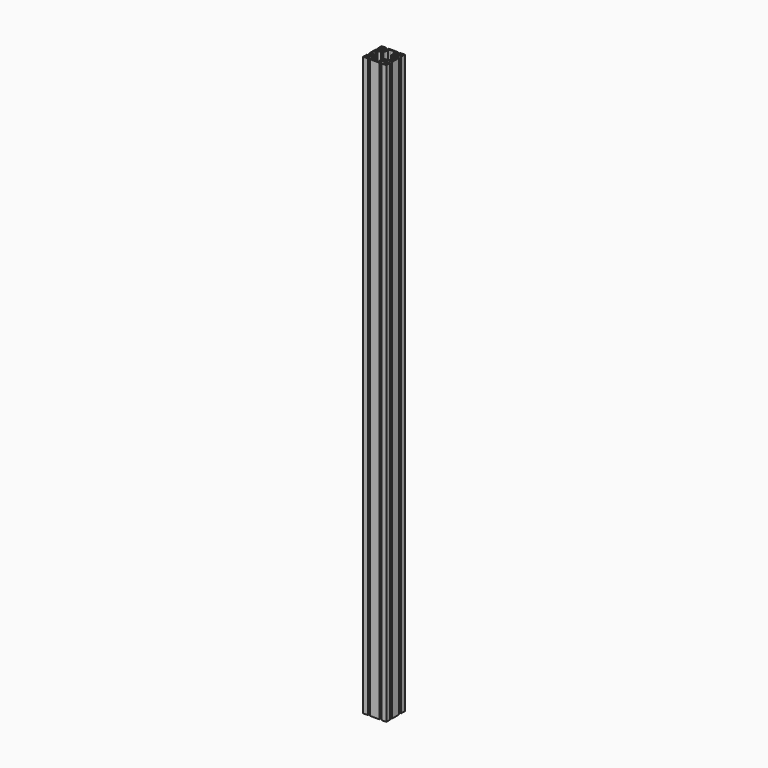
from build123d import *

# Parameters (mm, degrees)
F0_R     = 3
F0_R_2   = 2.5
F1_DEPTH = 1500
F2_R     = 2
F3_R     = 7


# Not quite as in the source:
# - a feature names something its author has since deleted; it is built from what else it names


with BuildPart() as f1:
    # F0 (on Top) → F1 (new body)
    with BuildSketch(Plane.XY):
        with BuildLine():
            Line((18.15, -30), (30, -30))
            Line((30, -30), (30, -18.15))
            Line((30, -18.15), (27.5, -18.15))
            Line((27.5, -18.15), (27.5, -20.15))
            Line((27.5, -20.15), (21.5477069044, -20.15))
            ThreePointArc((21.5477069044, -20.15), (19.5, -15), (21.5477069044, -9.85))
            Line((21.5477069044, -9.85), (27.5, -9.85))
            Line((27.5, -9.85), (27.5, -11.85))
            Line((27.5, -11.85), (30, -11.85))
            Line((30, -11.85), (30, 11.85))
            Line((30, 11.85), (27.5, 11.85))
            Line((27.5, 11.85), (27.5, 9.85))
            Line((27.5, 9.85), (21.5477069044, 9.85))
            ThreePointArc((21.5477069044, 9.85), (19.5, 15), (21.5477069044, 20.15))
            Line((21.5477069044, 20.15), (27.5, 20.15))
            Line((27.5, 20.15), (27.5, 18.15))
            Line((27.5, 18.15), (30, 18.15))
            Line((30, 18.15), (30, 30))
            Line((30, 30), (18.15, 30))
            Line((18.15, 30), (18.15, 27.5))
            Line((18.15, 27.5), (20.15, 27.5))
            Line((20.15, 27.5), (20.15, 21.5477069044))
            ThreePointArc((20.15, 21.5477069044), (15, 19.5), (9.85, 21.5477069044))
            Line((9.85, 21.5477069044), (9.85, 27.5))
            Line((9.85, 27.5), (11.85, 27.5))
            Line((11.85, 27.5), (11.85, 30))
            Line((11.85, 30), (-11.85, 30))
            Line((-11.85, 30), (-11.85, 27.5))
            Line((-11.85, 27.5), (-9.85, 27.5))
            Line((-9.85, 27.5), (-9.85, 21.5477069044))
            ThreePointArc((-9.85, 21.5477069044), (-15, 19.5), (-20.15, 21.5477069044))
            Line((-20.15, 21.5477069044), (-20.15, 27.5))
            Line((-20.15, 27.5), (-18.15, 27.5))
            Line((-18.15, 27.5), (-18.15, 30))
            Line((-18.15, 30), (-30, 30))
            Line((-30, 30), (-30, 18.15))
            Line((-30, 18.15), (-27.5, 18.15))
            Line((-27.5, 18.15), (-27.5, 20.15))
            Line((-27.5, 20.15), (-21.5477069044, 20.15))
            ThreePointArc((-21.5477069044, 20.15), (-19.5, 15), (-21.5477069044, 9.85))
            Line((-21.5477069044, 9.85), (-27.5, 9.85))
            Line((-27.5, 9.85), (-27.5, 11.85))
            Line((-27.5, 11.85), (-30, 11.85))
            Line((-30, 11.85), (-30, -11.85))
            Line((-30, -11.85), (-27.5, -11.85))
            Line((-27.5, -11.85), (-27.5, -9.85))
            Line((-27.5, -9.85), (-21.5477069044, -9.85))
            ThreePointArc((-21.5477069044, -9.85), (-19.5, -15), (-21.5477069044, -20.15))
            Line((-21.5477069044, -20.15), (-27.5, -20.15))
            Line((-27.5, -20.15), (-27.5, -18.15))
            Line((-27.5, -18.15), (-30, -18.15))
            Line((-30, -18.15), (-30, -30))
            Line((-30, -30), (-18.15, -30))
            Line((-18.15, -30), (-18.15, -27.5))
            Line((-18.15, -27.5), (-20.15, -27.5))
            Line((-20.15, -27.5), (-20.15, -21.5477069044))
            ThreePointArc((-20.15, -21.5477069044), (-15, -19.5), (-9.85, -21.5477069044))
            Line((-9.85, -21.5477069044), (-9.85, -27.5))
            Line((-9.85, -27.5), (-11.85, -27.5))
            Line((-11.85, -27.5), (-11.85, -30))
            Line((-11.85, -30), (11.85, -30))
            Line((11.85, -30), (11.85, -27.5))
            Line((11.85, -27.5), (9.85, -27.5))
            Line((9.85, -27.5), (9.85, -21.5477069044))
            ThreePointArc((9.85, -21.5477069044), (15, -19.5), (20.15, -21.5477069044))
            Line((20.15, -21.5477069044), (20.15, -27.5))
            Line((20.15, -27.5), (18.15, -27.5))
            Line((18.15, -27.5), (18.15, -30))
        make_face()
        with Locations((-25, -25)):
            Circle(F0_R, mode=Mode.SUBTRACT)
        with Locations((-15, -15)):
            Circle(F0_R_2, mode=Mode.SUBTRACT)
        with Locations((25, -25)):
            Circle(F0_R, mode=Mode.SUBTRACT)
        with Locations((15, -15)):
            Circle(F0_R_2, mode=Mode.SUBTRACT)
        with Locations((-25, 25)):
            Circle(F0_R, mode=Mode.SUBTRACT)
        with Locations((-15, 15)):
            Circle(F0_R_2, mode=Mode.SUBTRACT)
        Polygon((-7, 22), (-7, 27.5), (0, 27.5), (7, 27.5), (7, 22), (10, 16), (10, 10), (16, 10), (22, 7), (27.5, 7), (27.5, 0), (27.5, -7), (22, -7), (16, -10), (10, -10), (10, -16), (7, -22), (7, -27.5), (0, -27.5), (-7, -27.5), (-7, -22), (-10, -16), (-10, -10), (-16, -10), (-22, -7), (-27.5, -7), (-27.5, 0), (-27.5, 7), (-22, 7), (-16, 10), (-10, 10), (-10, 16), align=None, mode=Mode.SUBTRACT)
        with Locations((15, 15)):
            Circle(F0_R_2, mode=Mode.SUBTRACT)
        with Locations((25, 25)):
            Circle(F0_R, mode=Mode.SUBTRACT)
    extrude(amount=F1_DEPTH)

    # F2
    f2_edges = [f1.edges().sort_by_distance(p)[0] for p in [
        (-7, 27.5, 750),
        (7, 27.5, 750),
    ]]
    fillet(f2_edges, radius=F2_R)

    # F3
    f3_edges = [f1.edges().sort_by_distance(p)[0] for p in [
        (-10, 16, 750),
        (10, 16, 750),
    ]]
    fillet(f3_edges, radius=F3_R)


solid = f1.part
